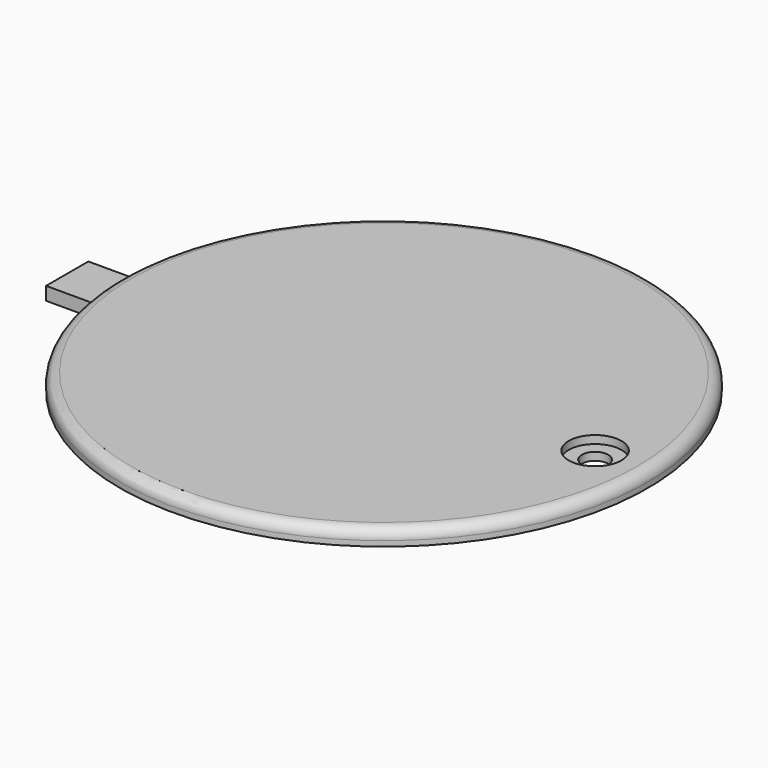
from build123d import *

# Parameters (mm, degrees)
F0_R     = 5
F1_DEPTH = 3
F0_R_2   = 2.5
F2_DEPTH = 1.5
F3_DEPTH = 2.5
F4_R     = 2.49999
F5_R     = 2


# Not quite as in the source:
# - a fillet or chamfer is up to 0.001 mm smaller than in the source, because OpenCascade refuses the exact size


with BuildPart() as f1:
    # F0 (on Top) → F1 (new body)
    with BuildSketch(Plane.XY):
        with BuildLine():
            ThreePointArc((-49.7493718553, -5), (2.503138753, -49.9373036555), (50, 0))
            ThreePointArc((50, 0), (2.503138753, 49.9373036555), (-49.7493718553, 5))
            Line((-49.7493718553, 5), (-40, 5))
            Line((-40, 5), (-40, -5))
            Line((-40, -5), (-49.7493718553, -5))
        make_face()
        with Locations((40, 0)):
            Circle(F0_R, mode=Mode.SUBTRACT)
        with BuildLine():
            Line((-40, 5), (-49.7493718553, 5))
            ThreePointArc((-49.7493718553, 5), (-50, 0), (-49.7493718553, -5))
            Line((-49.7493718553, -5), (-40, -5))
            Line((-40, -5), (-40, 5))
        make_face()
    extrude(amount=F1_DEPTH)

    # F0 (on Top) → F2 (join)
    with BuildSketch(Plane.XY):
        with Locations((40, 0)):
            Circle(F0_R)
        with Locations((40, 0)):
            Circle(F0_R_2, mode=Mode.SUBTRACT)
    extrude(amount=F2_DEPTH)

    # F0 (on Top) → F3 (join)
    with BuildSketch(Plane.XY):
        with BuildLine():
            ThreePointArc((-49.7493718553, -5), (-50, 0), (-49.7493718553, 5))
            Line((-49.7493718553, 5), (-60, 5))
            Line((-60, 5), (-60, -5))
            Line((-60, -5), (-49.7493718553, -5))
        make_face()
        with BuildLine():
            Line((-40, 5), (-49.7493718553, 5))
            ThreePointArc((-49.7493718553, 5), (-50, 0), (-49.7493718553, -5))
            Line((-49.7493718553, -5), (-40, -5))
            Line((-40, -5), (-40, 5))
        make_face()
    extrude(amount=-F3_DEPTH)

    # F4 (radius 2.5 in the source; OpenCascade refuses exactly that, so slightly less here)
    f4_edges = [f1.edges().sort_by_distance(p)[0] for p in [
        (-40, 0, -2.5),
    ]]
    fillet(f4_edges, radius=F4_R)

    # F5
    f5_edges = [f1.edges().sort_by_distance(p)[0] for p in [
        (-50, 0, 3),
    ]]
    fillet(f5_edges, radius=F5_R)


solid = f1.part
